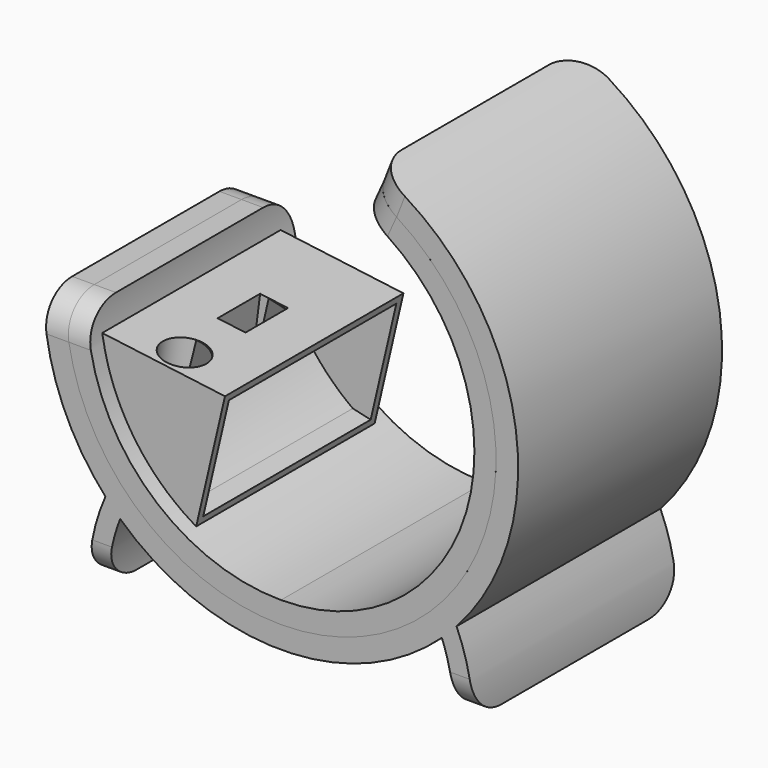
from build123d import *

# Parameters (mm, degrees)
F1_DEPTH      = 80
F2_DEPTH      = 80
F3_R          = 11.1053823869
F3_2_R        = 11.1053823869
F6_DEPTH      = 35
F6_DEPTH_BACK = 35
F8_DEPTH      = 26
F7_W          = 8.815
F7_H          = 16.672
F9_DEPTH      = 26
F10_W         = 65.713
F10_H         = 35.643
F11_DEPTH     = 21


with BuildPart() as f1:
    # F0 (on Front) → F1 (new body)
    with BuildSketch(Plane.XZ):
        with BuildLine():
            Line((0, -67.503), (0, -60.713))
            ThreePointArc((0, -60.713), (-42.9305740062, -42.9305740062), (-60.713, 0))
            Line((-60.713, 0), (-67.503, 0))
            ThreePointArc((-67.503, 0), (-47.7318290504, -47.7318290504), (0, -67.503))
        make_face()
        with BuildLine():
            Line((26.4210219705, 62.1175064457), (23.6194665166, 55.9302169714))
            ThreePointArc((23.6194665166, 55.9302169714), (59.505292336, -12.0494212727), (0, -60.713))
            Line((0, -60.713), (0, -67.503))
            ThreePointArc((0, -67.503), (66.1429249678, -13.4821543419), (26.4210219705, 62.1175064457))
        make_face()
    extrude(amount=F1_DEPTH)

    # F3
    f3_edges = [f1.edges().sort_by_distance(p)[0] for p in [
        (-64.108, -80, 0),
        (-64.108, 0, 0),
        (25.020244, -80, 59.023862),
        (25.020244, 0, 59.023862),
    ]]
    fillet(f3_edges, radius=F3_R)


with BuildPart() as f2:
    # F0 (on Front) → F2 (new body)
    with BuildSketch(Plane.XZ):
        with BuildLine():
            Line((0, -74.443), (0, -67.503))
            ThreePointArc((0, -67.503), (-47.7318290504, -47.7318290504), (-67.503, 0))
            Line((-67.503, 0), (-74.443, 0))
            ThreePointArc((-74.443, 0), (-69.4406504587, -26.8282745041), (-55.1058880387, -50.0509875274))
            ThreePointArc((-55.1058880387, -50.0509875274), (-52.8479074613, -52.4295615656), (-50.4873535385, -54.7063742326))
            ThreePointArc((-50.4873535385, -54.7063742326), (-27.104, -69.3334943083), (0, -74.443))
        make_face()
        with BuildLine():
            Line((28.9509467911, 68.5828180297), (26.4210219705, 62.1175064457))
            ThreePointArc((26.4210219705, 62.1175064457), (66.1429249678, -13.4821543419), (0, -67.503))
            Line((0, -67.503), (0, -74.443))
            ThreePointArc((0, -74.443), (27.104, -69.3334943083), (50.4873535385, -54.7063742326))
            ThreePointArc((50.4873535385, -54.7063742326), (52.8479074613, -52.4295615656), (55.1058880387, -50.0509875274))
            ThreePointArc((55.1058880387, -50.0509875274), (72.6971995722, 16.0273960255), (28.9509467911, 68.5828180297))
        make_face()
        with BuildLine():
            ThreePointArc((-54.208, -74.443), (-53.2697180611, -64.4008686678), (-50.4873535385, -54.7063742326))
            ThreePointArc((-50.4873535385, -54.7063742326), (-52.8479074613, -52.4295615656), (-55.1058880387, -50.0509875274))
            ThreePointArc((-55.1058880387, -50.0509875274), (-58.959627288, -61.9773865349), (-60.263, -74.443))
            Line((-60.263, -74.443), (-54.208, -74.443))
        make_face()
        with BuildLine():
            ThreePointArc((60.263, -74.443), (58.959627288, -61.9773865349), (55.1058880387, -50.0509875274))
            ThreePointArc((55.1058880387, -50.0509875274), (52.8479074613, -52.4295615656), (50.4873535385, -54.7063742326))
            ThreePointArc((50.4873535385, -54.7063742326), (53.2697180611, -64.4008686678), (54.208, -74.443))
            Line((54.208, -74.443), (60.263, -74.443))
        make_face()
    extrude(amount=F2_DEPTH)

    # F3#2
    f3_2_edges = [f2.edges().sort_by_distance(p)[0] for p in [
        (-70.973, -80, 0),
        (-70.973, 0, 0),
        (27.685984, -80, 65.350162),
        (27.685984, 0, 65.350162),
        (-57.2355, -80, -74.443),
        (-57.2355, 0, -74.443),
        (57.2355, -80, -74.443),
        (57.2355, 0, -74.443),
    ]]
    fillet(f3_2_edges, radius=F3_2_R)


with BuildPart() as f6:
    # F5 (on offset) → F6 (new body, two sides)
    with BuildSketch(Plane.XZ.offset(40)) as f6_sk:
        with BuildLine():
            Line((-21.5773568214, -13.4508206014), (-60.1168669908, -8.4870885591))
            ThreePointArc((-60.1168669908, -8.4870885591), (-50.4104761962, -33.8356654829), (-30.6281347583, -52.4212335817))
            Line((-30.6281347583, -52.4212335817), (-21.5773568214, -13.4508206014))
        make_face()
    extrude(amount=F6_DEPTH)
    extrude(f6_sk.sketch, amount=-F6_DEPTH_BACK)

    # F7 (on face) → F8 (cut)
    with BuildSketch(Plane(origin=(-2.0562349566, 0, -15.9650616406), x_dir=(0.9918075887, 0, -0.1277407805), z_dir=(0.1277407805, 0, 0.9918075887))):
        with BuildLine():
            ThreePointArc((-32.2202927461, -66.75), (-43.9839655752, -61.8773271708), (-39.1112927461, -73.641))
            ThreePointArc((-39.1112927461, -73.641), (-34.2386199169, -71.6226728292), (-32.2202927461, -66.75))
        make_face()
    extrude(amount=-F8_DEPTH, mode=Mode.SUBTRACT)

    # F7 (on face) → F9 (cut)
    with BuildSketch(Plane(origin=(-2.0562349566, 0, -15.9650616406), x_dir=(0.9918075887, 0, -0.1277407805), z_dir=(0.1277407805, 0, 0.9918075887))):
        with Locations((-39.1112927461, -40)):
            Rectangle(F7_W, F7_H)
    extrude(amount=-F9_DEPTH, mode=Mode.SUBTRACT)

    # F10 (on face) → F11 (cut)
    with BuildSketch(Plane(origin=(-17.5090216634, 0, 4.0664251377), x_dir=(0, 1, 0), z_dir=(0.9740747599, 0, -0.2262263515))):
        with Locations((-40, -37.987281626)):
            Rectangle(F10_W, F10_H)
    extrude(amount=-F11_DEPTH, mode=Mode.SUBTRACT)


solid = Compound([f1.part, f2.part, f6.part])
